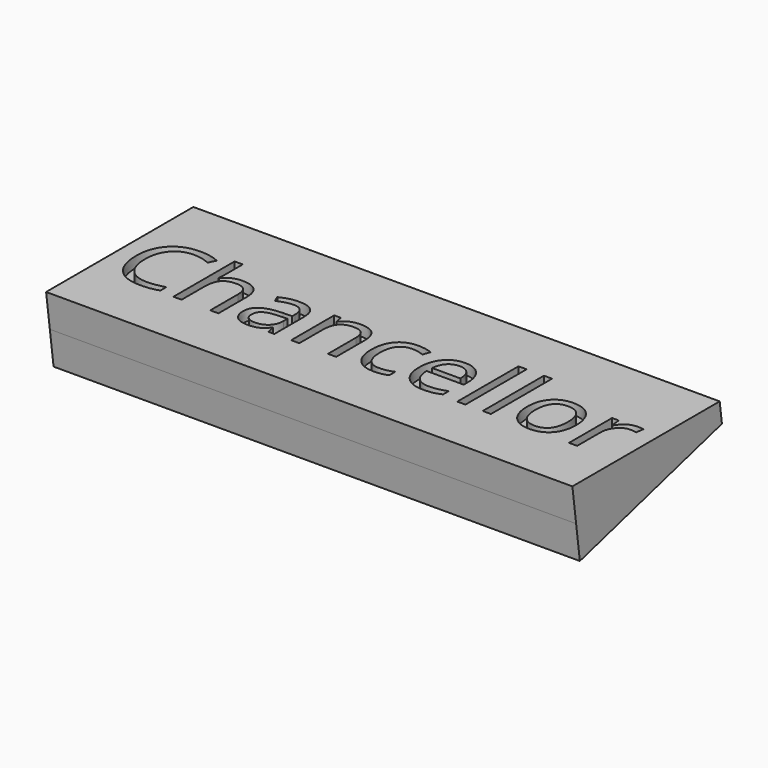
from build123d import *

# Parameters (mm, degrees)
F1_DEPTH      = 75
F1_DEPTH_BACK = 75
F2_TEXT_SIZE  = 28.6816880368
F3_DEPTH      = 3


# Not quite as in the source:
# - Text() gives the source's letters only with a copy of the font that has no kerning and outlines rounded to 1/6400 em; it was checked with that copy


with BuildPart() as f1:
    # F0 (on Right) → F1 (new body, two sides)
    with BuildSketch(Plane.YZ) as f1_sk:
        Polygon((-33.2611251304, 26.0748711193), (-31.927005009, 16.1642645031), (-30.5928848876, 6.2536578868), (20.0083854318, 20.1285071496), (19.6081493954, 23.1016891344), (19.2079133589, 26.0748711193), align=None)
    extrude(amount=F1_DEPTH)
    extrude(f1_sk.sketch, amount=-F1_DEPTH_BACK)

    # F2 (on face) → F3 (cut)
    with BuildSketch(Plane.XY.offset(26.0748711193)):
        with Locations((-72, -17.352013579)):
            Text('Chancellor', F2_TEXT_SIZE, font='Open Sans', text_align=(TextAlign.LEFT, TextAlign.BOTTOM))
    extrude(amount=-F3_DEPTH, mode=Mode.SUBTRACT)


solid = f1.part
